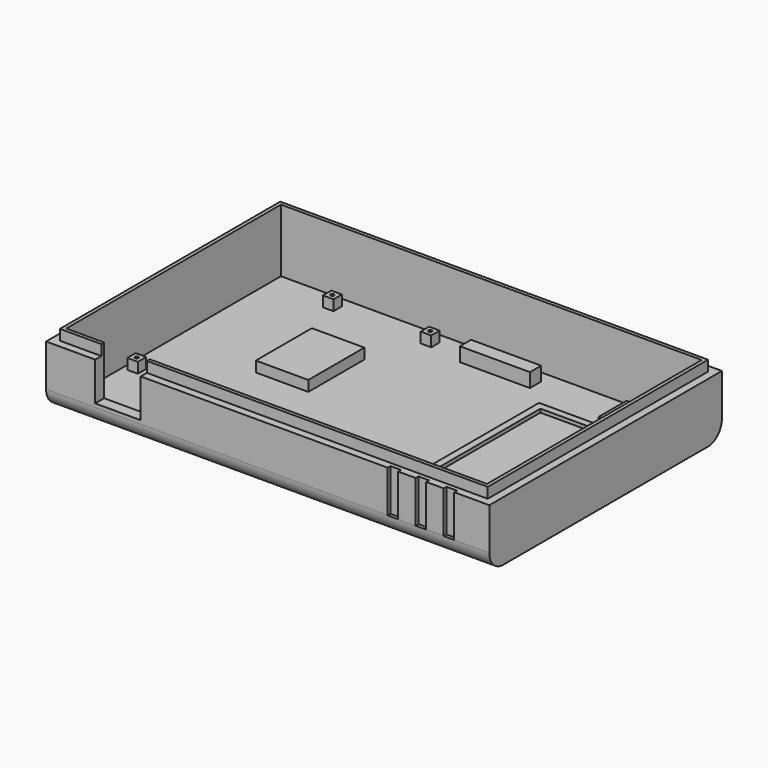
from build123d import *

# Parameters (mm, degrees)
F0_W      = 13
F0_H      = 0.2
F0_H_2    = 2
F1_DEPTH  = 17
F0_W_2    = 3
F0_H_3    = 3
F0_R      = 1.75
F0_H_4    = 1
F0_R_2    = 0.5
F2_DEPTH  = 2
F3_R      = 5
F5_DEPTH  = 3
F6_START  = 2
F6_DEPTH  = 18
F0_W_3    = 7.5
F0_H_5    = 20
F7_DEPTH  = 5
F8_W      = 13
F8_H      = 11
F8_H_2    = 3
F9_DEPTH  = 4
F8_W_2    = 3
F8_H_3    = 12
F10_DEPTH = 1
F4_W      = 3.3428409398
F4_H      = 12
F4_W_2    = 3
F11_DEPTH = 1
F12_DEPTH = 8
F13_DEPTH = 7
F14_DEPTH = 6
F16_DEPTH = 3


# Not quite as in the source:
# - a feature names something its author has since deleted; it is built from what else it names


with BuildPart() as f1:
    # F0 (on Top) → F1 (new body)
    with BuildSketch(Plane.XY):
        Polygon((63.25, -41.5), (63.25, 41.5), (11.25, 41.5), (-63.25, 41.5), (-63.25, -41.5), (-56.25, -41.5), (-56.25, -39.5), (-61.25, -39.5), (-61.25, 39.5), (61.25, 39.5), (61.25, -39.5), (-43.25, -39.5), (-43.25, -41.5), align=None)
        Polygon((-43.25, -39.3), (-43.25, -39.5), (61.25, -39.5), (61.25, 39.5), (-61.25, 39.5), (-61.25, -39.5), (-56.25, -39.5), (-56.25, -39.3), (-61.05, -39.3), (-61.05, 39.3), (61.05, 39.3), (61.05, -39.3), (-2.75, -39.3), align=None)
        with Locations((-49.75, -39.4)):
            Rectangle(F0_W, F0_H)
        with Locations((-49.75, -40.5)):
            Rectangle(F0_W, F0_H_2)
    extrude(amount=F1_DEPTH)

    # F0 (on Top) → F2 (join)
    with BuildSketch(Plane.XY):
        Polygon((-56.25, -38.3), (-43.25, -38.3), (60.05, -38.3), (60.05, 38.3), (-60.05, 38.3), (-60.05, -18.19), (-60.05, -38.3), align=None)
        Polygon((-58.55, -18.39), (-58.55, -18.19), (-58.55, -15.39), (-57.05, -15.39), (-55.55, -15.39), (-55.55, -18.39), align=None, mode=Mode.SUBTRACT)
        with Locations((-9.35, -18.19)):
            Rectangle(F0_W_2, F0_H_3, mode=Mode.SUBTRACT)
        Polygon((17, -30.19), (17, -34.19), (-3, -34.19), (-3, -30.19), (1, -30.19), (15, -30.19), align=None, mode=Mode.SUBTRACT)
        Polygon((-35.4, 18.51), (-27.9, 18.51), (-20.4, 18.51), (-20.4, -1.49), (-27.9, -1.49), (-35.4, -1.49), align=None, mode=Mode.SUBTRACT)
        Polygon((-43.35, 32.41), (-43.35, 33.91), (-43.35, 35.41), (-40.35, 35.41), (-40.35, 33.91), (-40.35, 32.41), align=None, mode=Mode.SUBTRACT)
        Polygon((-15.45, 32.41), (-15.45, 33.91), (-15.45, 35.41), (-12.45, 35.41), (-12.45, 32.41), align=None, mode=Mode.SUBTRACT)
        Polygon((51.25, -25), (24.25, -25), (24.25, 25), (36.25, 25), (41.25, 25), (41.25, 35), (53.25, 35), (53.25, 30), (53.25, 25), (53.25, -4), (57.25, -4), (59.25, -4), (59.25, -7), (57.25, -7), (53.25, -7), (53.25, -25), align=None, mode=Mode.SUBTRACT)
        Polygon((-3, 30.81), (-3, 34.81), (17, 34.81), (17, 30.81), (15, 30.81), (1, 30.81), align=None, mode=Mode.SUBTRACT)
        Polygon((-43.25, -38.3), (-43.25, -39.3), (-2.75, -39.3), (61.05, -39.3), (61.05, 39.3), (-61.05, 39.3), (-61.05, -39.3), (-56.25, -39.3), (-56.25, -38.3), (-60.05, -38.3), (-60.05, -18.19), (-60.05, 38.3), (60.05, 38.3), (60.05, -38.3), align=None)
        Polygon((41.25, 35), (41.25, 25), (51.25, 25), (53.25, 25), (53.25, 30), (53.25, 35), align=None)
        with Locations((49.42, 30)):
            Circle(F0_R, mode=Mode.SUBTRACT)
        Polygon((17, 34.81), (-3, 34.81), (-3, 30.81), (1, 30.81), (15, 30.81), (17, 30.81), align=None)
        with Locations((-49.75, -40.5)):
            Rectangle(F0_W, F0_H_2)
        Polygon((53.25, -4), (53.25, -7), (57.25, -7), (59.25, -7), (59.25, -4), (57.25, -4), align=None)
        with Locations((-49.75, -38.8)):
            Rectangle(F0_W, F0_H_4)
        with Locations((49.42, 30)):
            Circle(F0_R)
        with Locations((-9.35, -18.19)):
            Rectangle(F0_W_2, F0_H_3)
        with Locations((-9.35, -18.19)):
            Circle(F0_R_2, mode=Mode.SUBTRACT)
        with Locations((-49.75, -39.4)):
            Rectangle(F0_W, F0_H)
        with Locations((-9.35, -18.19)):
            Circle(F0_R_2)
    extrude(amount=F2_DEPTH)

    # F3
    f3_edges = [f1.edges().sort_by_distance(p)[0] for p in [
        (0, 41.5, 0),
        (0, -41.5, 0),
    ]]
    fillet(f3_edges, radius=F3_R)



with BuildPart() as f2:
    # F0 (on Top) → F2, piece 2 (new body)
    with BuildSketch(Plane.XY):
        with BuildLine():
            ThreePointArc((-57.05, -16.39), (-57.55, -16.89), (-57.05, -17.39))
            Line((-57.05, -17.39), (-57.05, -16.89))
            Line((-57.05, -16.89), (-57.05, -16.39))
        make_face()
        with BuildLine():
            Line((-57.05, -16.89), (-57.05, -17.39))
            ThreePointArc((-57.05, -17.39), (-56.6964466094, -17.2435533906), (-56.55, -16.89))
            ThreePointArc((-56.55, -16.89), (-56.6964466094, -16.5364466094), (-57.05, -16.39))
            Line((-57.05, -16.39), (-57.05, -16.89))
        make_face()
    extrude(amount=F2_DEPTH)


with BuildPart() as f2b:
    # F0 (on Top) → F2, piece 3 (new body)
    with BuildSketch(Plane.XY):
        with BuildLine():
            ThreePointArc((-13.45, 33.91), (-13.95, 34.41), (-14.45, 33.91))
            ThreePointArc((-14.45, 33.91), (-13.95, 33.41), (-13.45, 33.91))
        make_face()
    extrude(amount=F2_DEPTH)


with BuildPart() as f2c:
    # F0 (on Top) → F2, piece 4 (new body)
    with BuildSketch(Plane.XY):
        with BuildLine():
            ThreePointArc((-41.35, 33.91), (-41.85, 34.41), (-42.35, 33.91))
            Line((-42.35, 33.91), (-41.85, 33.91))
            Line((-41.85, 33.91), (-41.35, 33.91))
        make_face()
        with BuildLine():
            Line((-41.85, 33.91), (-42.35, 33.91))
            ThreePointArc((-42.35, 33.91), (-41.85, 33.41), (-41.35, 33.91))
            Line((-41.35, 33.91), (-41.85, 33.91))
        make_face()
    extrude(amount=F2_DEPTH)


with BuildPart() as f2d:
    # F0 (on Top) → F2, piece 5 (new body)
    with BuildSketch(Plane.XY):
        Polygon((51.25, 23), (26.25, 23), (26.25, -23), (49.25, -23), (51.25, -23), align=None)
    extrude(amount=F2_DEPTH)


with BuildPart() as f1_1:
    add(f1.part)

    add(f2d.part)  # F5 merges F2d
    # F0 (on Top) → F5 (join)
    with BuildSketch(Plane.XY):
        Polygon((24.25, 25), (24.25, -25), (51.25, -25), (53.25, -25), (53.25, -7), (53.25, -4), (53.25, 25), (51.25, 25), (41.25, 25), (36.25, 25), align=None)
        Polygon((26.25, -23), (26.25, 23), (51.25, 23), (51.25, -23), (49.25, -23), align=None, mode=Mode.SUBTRACT)
    extrude(amount=F5_DEPTH)

    # F0 (on Top) → F6 (join)
    with BuildSketch(Plane.XY.offset(F6_START)):
        Polygon((-43.25, -38.3), (-43.25, -39.3), (-2.75, -39.3), (61.05, -39.3), (61.05, 39.3), (-61.05, 39.3), (-61.05, -39.3), (-56.25, -39.3), (-56.25, -38.3), (-60.05, -38.3), (-60.05, -18.19), (-60.05, 38.3), (60.05, 38.3), (60.05, -38.3), align=None)
        with Locations((-49.75, -38.8)):
            Rectangle(F0_W, F0_H_4)
    extrude(amount=F6_DEPTH)


    add(f2.part)  # F7 merges F2

    add(f2b.part)  # F7 merges F2b

    add(f2c.part)  # F7 merges F2c
    # F0 (on Top) → F7 (join)
    with BuildSketch(Plane.XY):
        with Locations((-24.15, 8.51)):
            Rectangle(F0_W_3, F0_H_5)
        with Locations((-31.65, 8.51)):
            Rectangle(F0_W_3, F0_H_5)
        Polygon((41.25, 35), (41.25, 25), (51.25, 25), (53.25, 25), (53.25, 30), (53.25, 35), align=None)
        with Locations((49.42, 30)):
            Circle(F0_R, mode=Mode.SUBTRACT)
        with Locations((49.42, 30)):
            Circle(F0_R)
        Polygon((-15.45, 35.41), (-15.45, 33.91), (-15.45, 32.41), (-12.45, 32.41), (-12.45, 35.41), align=None)
        with BuildLine():
            ThreePointArc((-13.45, 33.91), (-13.95, 33.41), (-14.45, 33.91))
            ThreePointArc((-14.45, 33.91), (-13.95, 34.41), (-13.45, 33.91))
        make_face(mode=Mode.SUBTRACT)
        with Locations((-9.35, -18.19)):
            Rectangle(F0_W_2, F0_H_3)
        with Locations((-9.35, -18.19)):
            Circle(F0_R_2, mode=Mode.SUBTRACT)
        with BuildLine():
            Line((-57.05, -18.19), (-58.55, -18.19))
            Line((-58.55, -18.19), (-58.55, -18.39))
            Line((-58.55, -18.39), (-55.55, -18.39))
            Line((-55.55, -18.39), (-55.55, -15.39))
            Line((-55.55, -15.39), (-57.05, -15.39))
            Line((-57.05, -15.39), (-57.05, -16.39))
            ThreePointArc((-57.05, -16.39), (-56.6964466094, -16.5364466094), (-56.55, -16.89))
            ThreePointArc((-56.55, -16.89), (-56.6964466094, -17.2435533906), (-57.05, -17.39))
            Line((-57.05, -17.39), (-57.05, -18.19))
        make_face()
        with BuildLine():
            Line((-43.35, 35.41), (-43.35, 33.91))
            Line((-43.35, 33.91), (-42.35, 33.91))
            ThreePointArc((-42.35, 33.91), (-41.85, 34.41), (-41.35, 33.91))
            Line((-41.35, 33.91), (-40.35, 33.91))
            Line((-40.35, 33.91), (-40.35, 35.41))
            Line((-40.35, 35.41), (-43.35, 35.41))
        make_face()
        with BuildLine():
            Line((-42.35, 33.91), (-43.35, 33.91))
            Line((-43.35, 33.91), (-43.35, 32.41))
            Line((-43.35, 32.41), (-40.35, 32.41))
            Line((-40.35, 32.41), (-40.35, 33.91))
            Line((-40.35, 33.91), (-41.35, 33.91))
            ThreePointArc((-41.35, 33.91), (-41.85, 33.41), (-42.35, 33.91))
        make_face()
        with BuildLine():
            Line((-58.55, -15.39), (-58.55, -18.19))
            Line((-58.55, -18.19), (-57.05, -18.19))
            Line((-57.05, -18.19), (-57.05, -17.39))
            ThreePointArc((-57.05, -17.39), (-57.55, -16.89), (-57.05, -16.39))
            Line((-57.05, -16.39), (-57.05, -15.39))
            Line((-57.05, -15.39), (-58.55, -15.39))
        make_face()
    extrude(amount=F7_DEPTH)

    # F8 (on face) → F9 (cut)
    with BuildSketch(Plane.XZ.offset(41.5)):
        with Locations((-42.75, 11.5)):
            Rectangle(F8_W, F8_H)
        with Locations((-42.75, 18.5)):
            Rectangle(F8_W, F8_H_2)
    extrude(amount=-F9_DEPTH, mode=Mode.SUBTRACT)

    # F8 (on face) → F10 (cut)
    with BuildSketch(Plane.XZ.offset(41.5)):
        Polygon((-49.25, 20), (-49.25, 17), (-49.25, 6), (-36.25, 6), (-36.25, 20), align=None)
        with Locations((51.75, 11)):
            Rectangle(F8_W_2, F8_H_3)
        with Locations((35.75, 11)):
            Rectangle(F8_W_2, F8_H_3)
        with Locations((43.75, 11)):
            Rectangle(F8_W_2, F8_H_3)
    extrude(amount=-F10_DEPTH, mode=Mode.SUBTRACT)

    # F4 (on face) → F11 (cut)
    with BuildSketch(Plane(origin=(0, 41.5, 0), x_dir=(-1, 0, 0), z_dir=(0, 1, 0))):
        with Locations((-51.5785795301, 11)):
            Rectangle(F4_W, F4_H)
        with Locations((-43.4071590602, 11)):
            Rectangle(F4_W_2, F4_H)
        with Locations((-35.4071590602, 11)):
            Rectangle(F4_W_2, F4_H)
        with Locations((35.4071590602, 11)):
            Rectangle(F4_W_2, F4_H)
        with Locations((43.4071590602, 11)):
            Rectangle(F4_W_2, F4_H)
        with Locations((51.5785795301, 11)):
            Rectangle(F4_W, F4_H)
    extrude(amount=-F11_DEPTH, mode=Mode.SUBTRACT)

    # F0 (on Top) → F12 (join)
    with BuildSketch(Plane.XY):
        Polygon((53.25, -4), (53.25, -7), (57.25, -7), (59.25, -7), (59.25, -4), (57.25, -4), align=None)
    extrude(amount=F12_DEPTH)

    # F0 (on Top) → F13 (join)
    with BuildSketch(Plane.XY):
        with Locations((49.42, 30)):
            Circle(F0_R)
    extrude(amount=F13_DEPTH)

    # F0 (on Top) → F14 (join)
    with BuildSketch(Plane.XY):
        Polygon((17, 34.81), (-3, 34.81), (-3, 30.81), (1, 30.81), (15, 30.81), (17, 30.81), align=None)
        Polygon((-3, -34.19), (17, -34.19), (17, -30.19), (15, -30.19), (1, -30.19), (-3, -30.19), align=None)
    extrude(amount=F14_DEPTH)

    # F15 (on face) → F16 (cut)
    with BuildSketch(Plane.XZ.offset(7)):
        with BuildLine():
            ThreePointArc((56.25, 7), (54.8357864376, 3.5857864376), (58.25, 5))
            ThreePointArc((58.25, 5), (57.6642135624, 6.4142135624), (56.25, 7))
        make_face()
    extrude(amount=-F16_DEPTH, mode=Mode.SUBTRACT)


solid = f1_1.part
